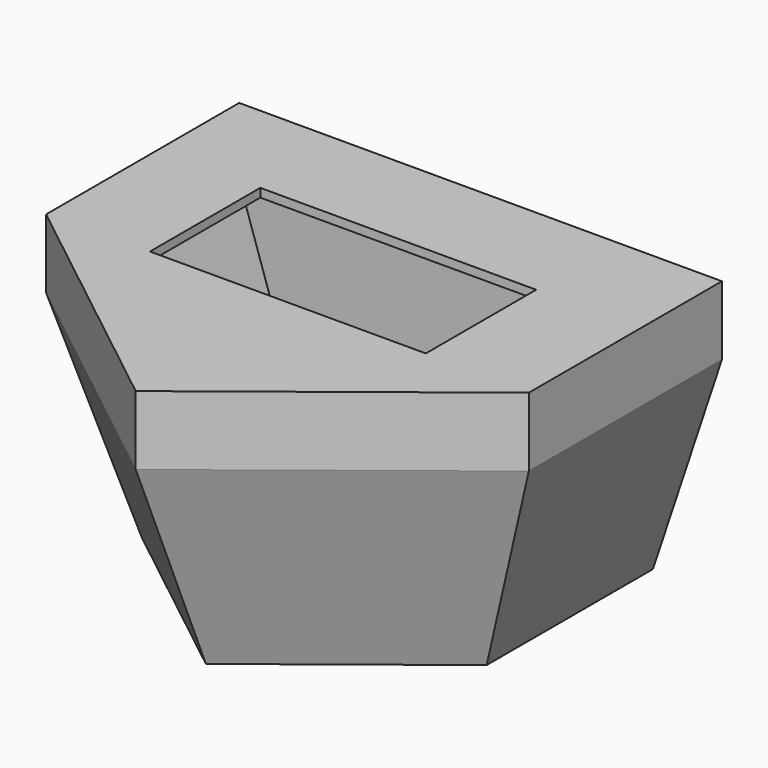
from build123d import *

# Parameters (mm, degrees)
F0_W         = 355.6
F0_H         = 177.8
F1_DEPTH     = 203.2
F2_C1_SIZE2  = 50.8
F2_C1_SIZE   = 152.4
F2_C2_SIZE2  = 152.4
F2_C2_SIZE   = 50.8
F6_DEPTH     = 50.8
F8_DEPTH     = 152.4
F9_T1_DEPTH  = 1017.0916674945
F10_T1_DEPTH = 964.80725191
F11_T        = -6.35
F13_W        = 203.2
F13_H        = 101.6
F14_DEPTH    = 6.35


# Not quite as in the source:
# - a fillet or chamfer that OpenCascade refuses, or shapes differently, is made with other operations: its cross-section is extruded or revolved along the edge and cut away or added
# - two fillets or chamfers of one size are made in one step


with BuildPart() as f1:
    # F0 (on Top) → F1 (new body)
    with BuildSketch(Plane.XY):
        Rectangle(F0_W, F0_H)
    extrude(amount=F1_DEPTH)

    # F2: chamfer of 50.8 x 152.4 on 2 edges, made by hand

    # F2_c1
    f2_c1_edges = [f1.edges().sort_by_distance(p)[0] for p in [
        (-177.8, 0, 0),
    ]]
    f2_c1_side = f1.faces().sort_by_distance((-177.8, 0, 1.016))[0]
    chamfer(f2_c1_edges, length=F2_C1_SIZE, length2=F2_C1_SIZE2, reference=f2_c1_side)

    # F2_c2
    f2_c2_edges = [f1.edges().sort_by_distance(p)[0] for p in [
        (177.8, 0, 0),
    ]]
    f2_c2_side = f1.faces().sort_by_distance((176.784, 0, 0))[0]
    chamfer(f2_c2_edges, length=F2_C2_SIZE, length2=F2_C2_SIZE2, reference=f2_c2_side)

    # F5 (on face) → F6 (join)
    with BuildSketch(Plane.XY.offset(203.2)):
        Polygon((0, -228.5999999986), (177.8, -88.9), (-177.8, -88.9), align=None)
    extrude(amount=-F6_DEPTH)

    # F7: union 

    # F8 (add): a face of the model
    f8_faces = [f1.faces().sort_by_distance(p)[0] for p in [
        (0, -135.4666666662, 152.4),
    ]]
    extrude(f8_faces, amount=F8_DEPTH)

    # F9: chamfer of 152.4 x 50.8 on 1 edges, made by hand

    # F9_s2 → F9_t1 (cut)
    with BuildSketch(Plane(origin=(-422.0338047977, -331.5979894806, 0), x_dir=(0, 0, 1), z_dir=(0.7863183388, 0.6178215519, 0))):
        Polygon((152.4, 179.7523722544), (0, 128.9523722544), (0, 179.7523722544), align=None)
    extrude(amount=F9_T1_DEPTH, mode=Mode.SUBTRACT)

    # F10: chamfer of 152.4 x 50.8 on 1 edges, made by hand

    # F10_s2 → F10_t1 (cut)
    with BuildSketch(Plane(origin=(-377.7240256197, 296.783162984, 0), x_dir=(0, 0, 1), z_dir=(0.7863183388, -0.6178215519, 0))):
        Polygon((0, 128.9523722544), (152.4, 179.7523722544), (0, 179.7523722544), align=None)
    extrude(amount=F10_T1_DEPTH, mode=Mode.SUBTRACT)

    # F11
    f11_openings = [f1.faces().sort_by_distance(p)[0] for p in [
        (0, -38.208547, 203.2),
    ]]
    offset(amount=F11_T, openings=f11_openings)

    # F13 (on face) → F14 (join)
    with BuildSketch(Plane(origin=(0, 0, 203.2), x_dir=(1, 0, 0), z_dir=(0, 0, -1))):
        Polygon((0, 228.5980195153), (-177.8, 88.899947989), (-177.8, -88.900052011), (177.8, -88.900052011), (177.8, 88.899947989), align=None)
        with Locations((-0.631964469, 36.9129354686)):
            Rectangle(F13_W, F13_H, mode=Mode.SUBTRACT)
    extrude(amount=F14_DEPTH)


solid = f1.part
